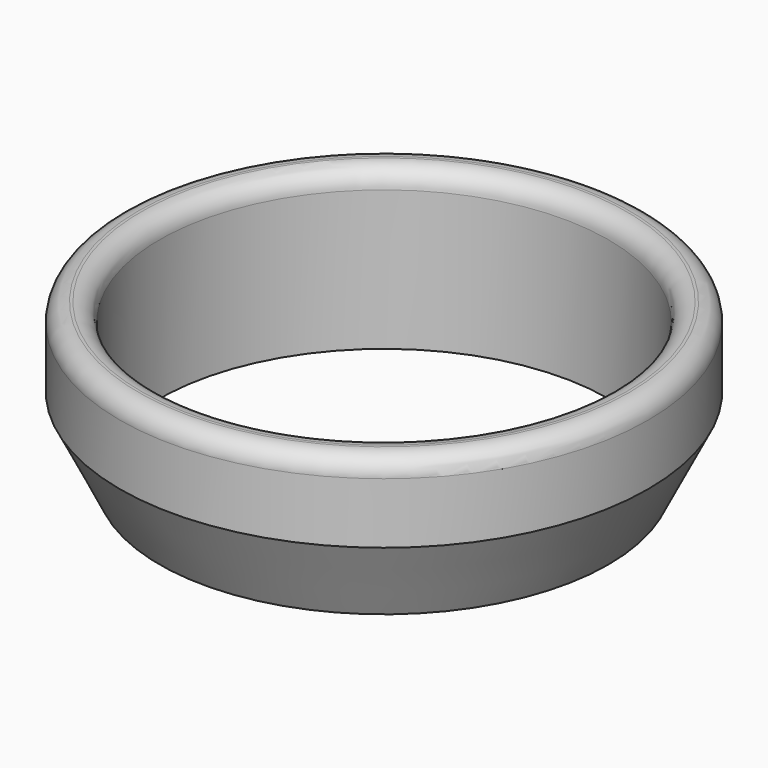
from build123d import *

# Parameters (mm, degrees)
F0_R     = 50
F0_R_2   = 42.5
F1_DEPTH = 15
F2_SIZE2 = 7.49999
F2_SIZE  = 14.99999
F3_R     = 3.5


# Not quite as in the source:
# - a fillet or chamfer is up to 0.001 mm smaller than in the source, because OpenCascade refuses the exact size


with BuildPart() as f1:
    # F0 (on Top) → F1 (new body, symmetric)
    with BuildSketch(Plane.XY):
        Circle(F0_R)
        Circle(F0_R_2, mode=Mode.SUBTRACT)
    extrude(amount=F1_DEPTH, both=True)

    # F2 (size 15 and 7.5 in the source; OpenCascade refuses exactly that, so slightly less here)
    f2_edges = [f1.edges().sort_by_distance(p)[0] for p in [
        (-50, 0, -15),
    ]]
    f2_side = f1.faces().sort_by_distance((-50, 0, 0))[0]
    chamfer(f2_edges, length=F2_SIZE, length2=F2_SIZE2, reference=f2_side)

    # F3
    f3_edges = [f1.edges().sort_by_distance(p)[0] for p in [
        (-50, 0, 15),
        (-42.5, 0, 15),
    ]]
    fillet(f3_edges, radius=F3_R)


solid = f1.part
